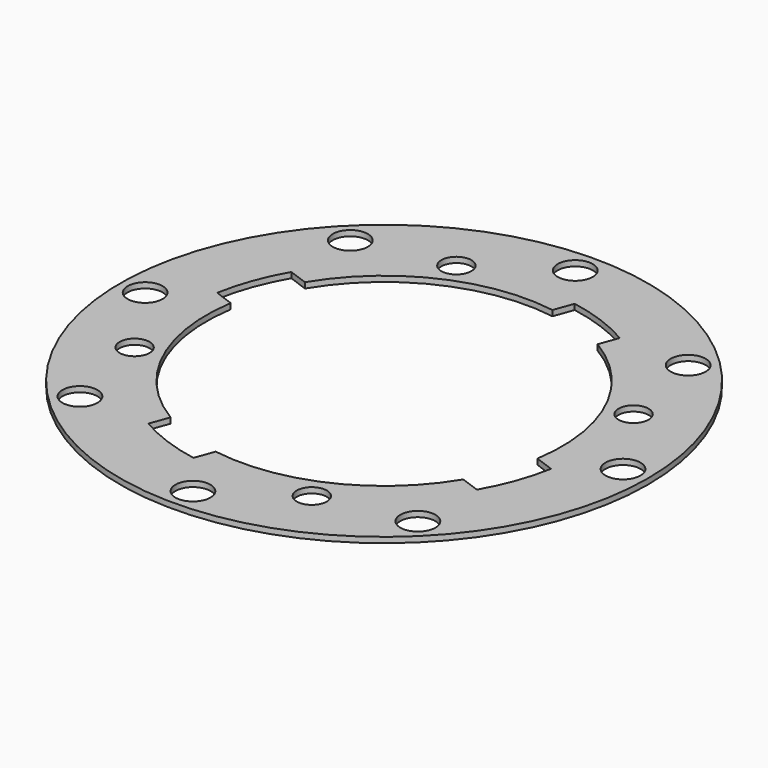
from build123d import *

# Parameters (mm, degrees)
F0_R            = 301.625
F0_R_2          = 17.145
F0_R_3          = 20.0025
F1_DEPTH        = 6.35
F2_DEPTH        = 6.351
F2_COPIES_COUNT = 8
F3_DEPTH        = 6.351
F3_COPIES_COUNT = 4
F4_DEPTH        = 6.351
F4_COPIES_COUNT = 4


# Not quite as in the source:
# - a pattern or mirror of a feature is missing from the dataset's text; its kind, count and spacing are read off the source's solid


with BuildPart() as f1:
    # F0 (on Top) → F1 (new body)
    with BuildSketch(Plane.XY):
        Circle(F0_R)
        with Locations((-88.6964525364, 214.1321786478)):
            Circle(F0_R_2, mode=Mode.SUBTRACT)
        with BuildLine():
            ThreePointArc((104.6230881005, 174.1960086693), (176.846899184, 100.0770415679), (203.2, 0))
            ThreePointArc((203.2, 0), (-154.5268592771, -131.9533620714), (31.8251007682, 200.6923091728))
            Line((31.8251007682, 200.6923091728), (39.7746000853, 222.5333790425))
            ThreePointArc((39.7746000853, 222.5333790425), (77.3170736002, 212.4269138549), (112.5725874176, 196.037078539))
            Line((112.5725874176, 196.037078539), (104.6230881005, 174.1960086693))
        make_face(mode=Mode.SUBTRACT)
        with Locations((0, 273.05)):
            Circle(F0_R_3, mode=Mode.SUBTRACT)
        with BuildLine():
            ThreePointArc((31.8251007682, 200.6923091728), (69.4984931238, 190.9455405437), (104.6230881005, 174.1960086693))
            Line((104.6230881005, 174.1960086693), (112.5725874176, 196.037078539))
            ThreePointArc((112.5725874176, 196.037078539), (77.3170736002, 212.4269138549), (39.7746000853, 222.5333790425))
            Line((39.7746000853, 222.5333790425), (31.8251007682, 200.6923091728))
        make_face()
        with Locations((0, 273.05)):
            Circle(F0_R_3)
        with Locations((-88.6964525364, 214.1321786478)):
            Circle(F0_R_2)
    extrude(amount=F1_DEPTH)

    # F0 (on Top) → F2 (cut, through all)
    with BuildSketch(Plane.XY):
        with Locations((0, 273.05)):
            Circle(F0_R_3)
    f2 = extrude(amount=F2_DEPTH, mode=Mode.SUBTRACT)

    # F2_copies: F2 ×8 about axis
    f2_copies_axis = Axis((0, 0, 0), (0, 0, 1))
    for i in range(1, F2_COPIES_COUNT):
        add(f2.rotate(f2_copies_axis, i * 360 / F2_COPIES_COUNT), mode=Mode.SUBTRACT)

    # F0 (on Top) → F3 (cut, through all)
    with BuildSketch(Plane.XY):
        with BuildLine():
            ThreePointArc((31.8251007682, 200.6923091728), (69.4984931238, 190.9455405437), (104.6230881005, 174.1960086693))
            Line((104.6230881005, 174.1960086693), (112.5725874176, 196.037078539))
            ThreePointArc((112.5725874176, 196.037078539), (77.3170736002, 212.4269138549), (39.7746000853, 222.5333790425))
            Line((39.7746000853, 222.5333790425), (31.8251007682, 200.6923091728))
        make_face()
    f3 = extrude(amount=F3_DEPTH, mode=Mode.SUBTRACT)

    # F3_copies: F3 ×4 about axis
    f3_copies_axis = Axis((0, 0, 0), (0, 0, 1))
    for i in range(1, F3_COPIES_COUNT):
        add(f3.rotate(f3_copies_axis, i * 360 / F3_COPIES_COUNT), mode=Mode.SUBTRACT)

    # F0 (on Top) → F4 (cut, through all)
    with BuildSketch(Plane.XY):
        with Locations((-88.6964525364, 214.1321786478)):
            Circle(F0_R_2)
    f4 = extrude(amount=F4_DEPTH, mode=Mode.SUBTRACT)

    # F4_copies: F4 ×4 about axis
    f4_copies_axis = Axis((0, 0, 0), (0, 0, 1))
    for i in range(1, F4_COPIES_COUNT):
        add(f4.rotate(f4_copies_axis, i * 360 / F4_COPIES_COUNT), mode=Mode.SUBTRACT)


solid = f1.part
